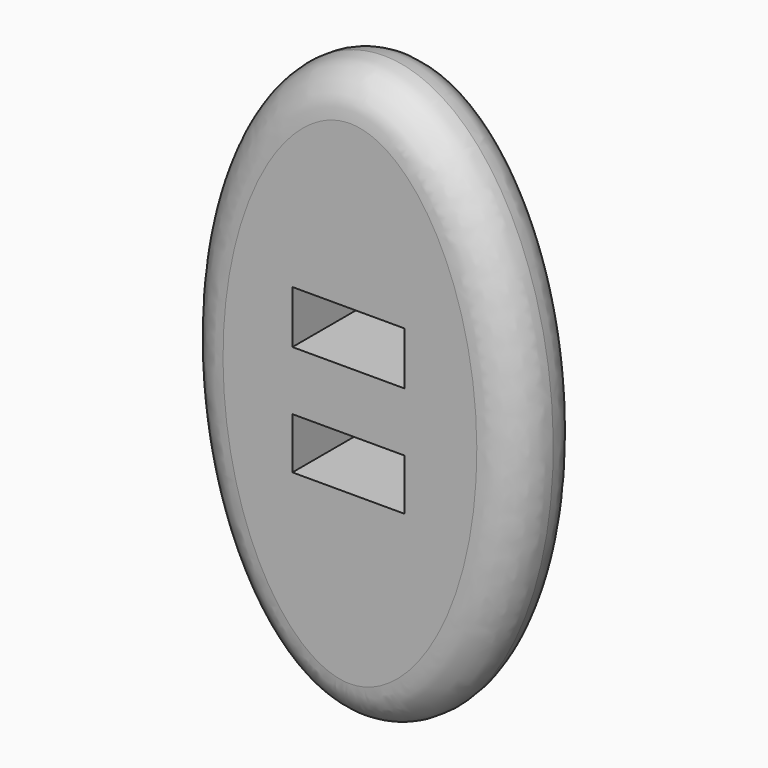
from build123d import *

# Parameters (mm, degrees)
F1_DEPTH = 12.7
F2_R     = 6.35
F3_R     = 6.34999
F4_W     = 16.7462797835
F4_H     = 7.9079647548
F4_H_2   = 7.675377652
F5_DEPTH = 25.4


# Not quite as in the source:
# - a fillet or chamfer is up to 0.001 mm smaller than in the source, because OpenCascade refuses the exact size


with BuildPart() as f1:
    # F0 (on Front) → F1 (new body)
    with BuildSketch(Plane.XZ):
        with BuildLine():
            add(Edge.make_bspline(
                [(0, -43.2612225413), (43.8914086801, -43.2612225413), (21.9457043401, 21.6306112707), (0, 86.5224450827), (-21.9457043401, 21.6306112707), (-43.8914086801, -43.2612225413), (0, -43.2612225413)],
                knots=[0, 0, 0, 2.0943951024, 2.0943951024, 4.1887902048, 4.1887902048, 6.2831853072, 6.2831853072, 6.2831853072], degree=2, weights=[1, 0.5, 1, 0.5, 1, 0.5, 1]))
        make_face()
    extrude(amount=F1_DEPTH)

    # F2
    f2_edges = [f1.edges().sort_by_distance(p)[0] for p in [
        (1e-06, 0, 43.261223),
    ]]
    fillet(f2_edges, radius=F2_R)

    # F3 (radius 6.35 in the source; OpenCascade refuses exactly that, so slightly less here)
    f3_edges = [f1.edges().sort_by_distance(p)[0] for p in [
        (1e-06, -12.7, 43.261223),
    ]]
    fillet(f3_edges, radius=F3_R)

    # F4 (on face) → F5 (cut)
    with BuildSketch(Plane(origin=(0, 0, 0), x_dir=(-1, 0, 0), z_dir=(0, 1, 0))):
        with Locations((0.2325871028, 8.6057267617)):
            Rectangle(F4_W, F4_H)
        with Locations((0.2325871028, -8.0242585391)):
            Rectangle(F4_W, F4_H_2)
    extrude(amount=-F5_DEPTH, mode=Mode.SUBTRACT)


solid = f1.part
